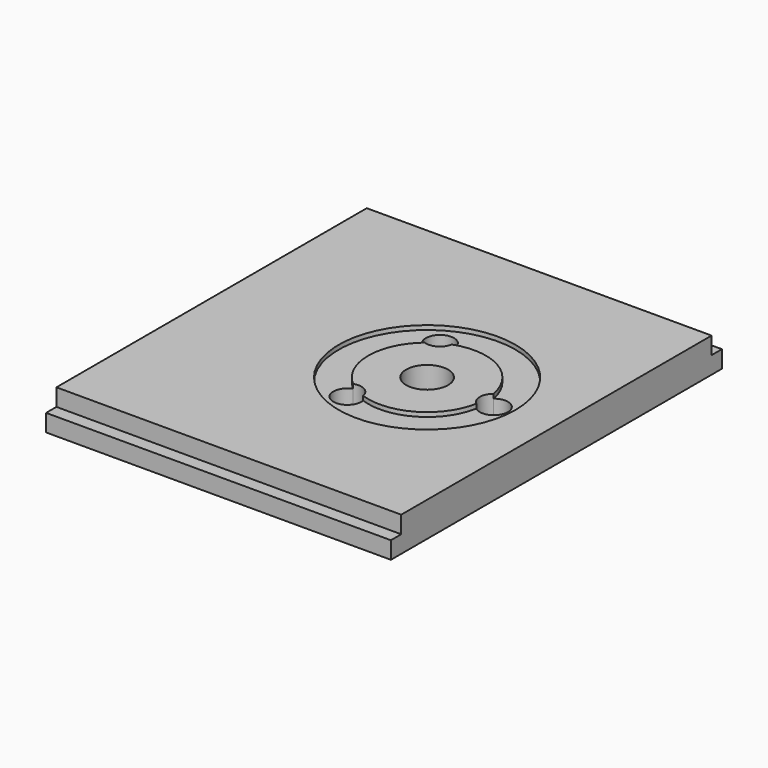
from build123d import *

# Parameters (mm, degrees)
F0_W     = 80
F0_H     = 96
F0_R     = 20.5
F1_DEPTH = 8
F0_R_2   = 4.8708945169
F2_DEPTH = 7
F0_R_3   = 1.5
F3_DEPTH = 3
F4_R     = 2.5
F5_DEPTH = 25
F6_W     = 3
F6_H     = 9.6463483796
F6_H_2   = 12.8309304863
F7_DEPTH = 100


# Not quite as in the source:
# - a feature names something its author has since deleted; it is built from what else it names


with BuildPart() as f1:
    # F0 (on Top) → F1 (new body)
    with BuildSketch(Plane.XY):
        with Locations((-10, 0)):
            Rectangle(F0_W, F0_H)
        Circle(F0_R, mode=Mode.SUBTRACT)
    extrude(amount=F1_DEPTH)



with BuildPart() as f1b:
    # F0 (on Top) → F1, piece 2 (new body)
    with BuildSketch(Plane.XY):
        with BuildLine():
            ThreePointArc((13.4196774194, -2.4969497313), (12.25, 0), (13.4196774194, 2.4969497313))
            ThreePointArc((13.4196774194, 2.4969497313), (6.825, 11.8212467617), (-4.5474168104, 12.8702564214))
            ThreePointArc((-4.5474168104, 12.8702564214), (-6.125, 10.6088111964), (-8.8722606089, 10.3733066901))
            ThreePointArc((-8.8722606089, 10.3733066901), (-13.65, 0), (-8.8722606089, -10.3733066901))
            ThreePointArc((-8.8722606089, -10.3733066901), (-6.125, -10.6088111964), (-4.5474168104, -12.8702564214))
            ThreePointArc((-4.5474168104, -12.8702564214), (6.825, -11.8212467617), (13.4196774194, -2.4969497313))
        make_face()
        Circle(F0_R_2, mode=Mode.SUBTRACT)
    extrude(amount=F1_DEPTH)


with BuildPart() as f1_1:
    add(f1.part)

    add(f1b.part)  # F2 merges F1b
    # F0 (on Top) → F2 (join)
    with BuildSketch(Plane.XY):
        Circle(F0_R)
        with BuildLine():
            ThreePointArc((-4.5474168104, 12.8702564214), (6.825, 11.8212467617), (13.4196774194, 2.4969497313))
            ThreePointArc((13.4196774194, 2.4969497313), (16.8786681277, 2.9430892262), (18.75, 0))
            ThreePointArc((18.75, 0), (16.8786681277, -2.9430892262), (13.4196774194, -2.4969497313))
            ThreePointArc((13.4196774194, -2.4969497313), (6.825, -11.8212467617), (-4.5474168104, -12.8702564214))
            ThreePointArc((-4.5474168104, -12.8702564214), (-4.5118759006, -13.1458107676), (-4.5, -13.4233937587))
            ThreePointArc((-4.5, -13.4233937587), (-9.6094559716, -16.0888999938), (-8.8722606089, -10.3733066901))
            ThreePointArc((-8.8722606089, -10.3733066901), (-13.65, 0), (-8.8722606089, 10.3733066901))
            ThreePointArc((-8.8722606089, 10.3733066901), (-9.6094559716, 16.0888999938), (-4.5, 13.4233937587))
            ThreePointArc((-4.5, 13.4233937587), (-4.5118759006, 13.1458107676), (-4.5474168104, 12.8702564214))
        make_face(mode=Mode.SUBTRACT)
    extrude(amount=F2_DEPTH)

    # F0 (on Top) → F3 (join)
    with BuildSketch(Plane.XY):
        with BuildLine():
            ThreePointArc((-4.5, -13.4233937587), (-4.5118759006, -13.1458107676), (-4.5474168104, -12.8702564214))
            ThreePointArc((-4.5474168104, -12.8702564214), (-6.825, -11.8212467617), (-8.8722606089, -10.3733066901))
            ThreePointArc((-8.8722606089, -10.3733066901), (-9.6094559716, -16.0888999938), (-4.5, -13.4233937587))
        make_face()
        with Locations((-7.75, -13.4233937587)):
            Circle(F0_R_3, mode=Mode.SUBTRACT)
        with BuildLine():
            ThreePointArc((-8.8722606089, -10.3733066901), (-6.825, -11.8212467617), (-4.5474168104, -12.8702564214))
            ThreePointArc((-4.5474168104, -12.8702564214), (-6.125, -10.6088111964), (-8.8722606089, -10.3733066901))
        make_face()
        with BuildLine():
            ThreePointArc((13.4196774194, 2.4969497313), (13.5922973918, 1.2537749451), (13.65, 0))
            ThreePointArc((13.65, 0), (13.5922973918, -1.2537749451), (13.4196774194, -2.4969497313))
            ThreePointArc((13.4196774194, -2.4969497313), (16.8786681277, -2.9430892262), (18.75, 0))
            ThreePointArc((18.75, 0), (16.8786681277, 2.9430892262), (13.4196774194, 2.4969497313))
        make_face()
        with Locations((15.5, 0)):
            Circle(F0_R_3, mode=Mode.SUBTRACT)
        with BuildLine():
            ThreePointArc((13.4196774194, -2.4969497313), (13.5922973918, -1.2537749451), (13.65, 0))
            ThreePointArc((13.65, 0), (13.5922973918, 1.2537749451), (13.4196774194, 2.4969497313))
            ThreePointArc((13.4196774194, 2.4969497313), (12.25, 0), (13.4196774194, -2.4969497313))
        make_face()
        with BuildLine():
            ThreePointArc((-8.8722606089, 10.3733066901), (-6.825, 11.8212467617), (-4.5474168104, 12.8702564214))
            ThreePointArc((-4.5474168104, 12.8702564214), (-4.5118759006, 13.1458107676), (-4.5, 13.4233937587))
            ThreePointArc((-4.5, 13.4233937587), (-9.6094559716, 16.0888999938), (-8.8722606089, 10.3733066901))
        make_face()
        with Locations((-7.75, 13.4233937587)):
            Circle(F0_R_3, mode=Mode.SUBTRACT)
        with BuildLine():
            ThreePointArc((-8.8722606089, 10.3733066901), (-6.125, 10.6088111964), (-4.5474168104, 12.8702564214))
            ThreePointArc((-4.5474168104, 12.8702564214), (-6.825, 11.8212467617), (-8.8722606089, 10.3733066901))
        make_face()
    extrude(amount=F3_DEPTH)

    # F4 (on face) → F5 (cut)
    with BuildSketch(Plane(origin=(-50, 0, 0), x_dir=(0, -1, 0), z_dir=(-1, 0, 0))):
        with Locations((0, 4)):
            Circle(F4_R)
    extrude(amount=-F5_DEPTH, mode=Mode.SUBTRACT)

    # F6 (on face) → F7 (cut)
    with BuildSketch(Plane(origin=(-50, 0, 0), x_dir=(0, -1, 0), z_dir=(-1, 0, 0))):
        with Locations((46.5, 8.8231741898)):
            Rectangle(F6_W, F6_H)
        with Locations((-46.5, 10.4154652432)):
            Rectangle(F6_W, F6_H_2)
    extrude(amount=-F7_DEPTH, mode=Mode.SUBTRACT)


solid = f1_1.part
